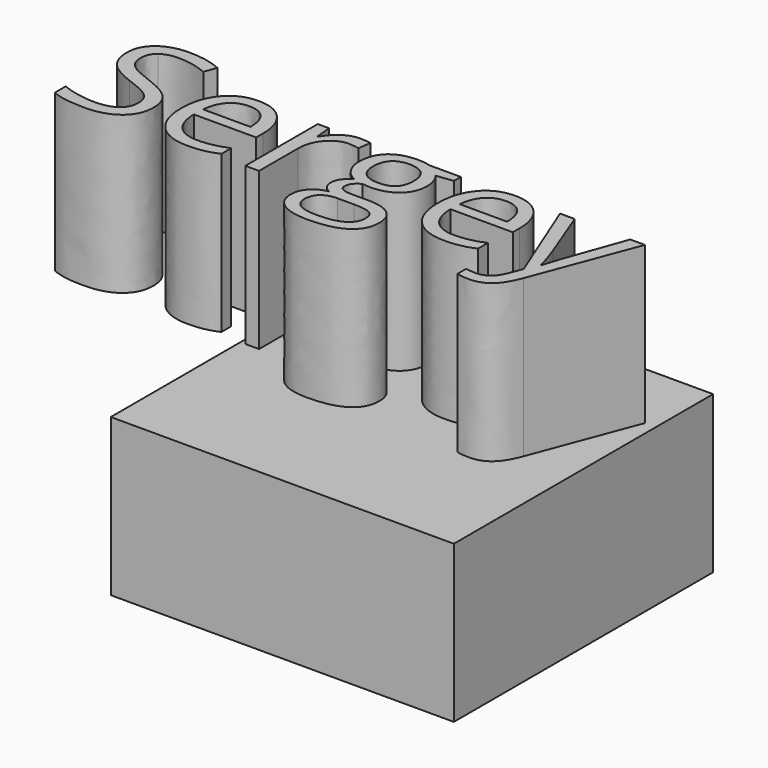
from build123d import *

# Parameters (mm, degrees)
F0_W         = 55.5511265993
F0_H         = 52.472114563
F1_DEPTH     = 25.4
F2_TEXT_SIZE = 27.3882670121
F4_DEPTH     = 25.4
F6_DEPTH     = 25.4


# Not quite as in the source:
# - Text() gives the source's letters only with a copy of the font that has no kerning and outlines rounded to 1/6400 em; it was checked with that copy


with BuildPart() as f1:
    # F0 (on Top) → F1 (new body)
    with BuildSketch(Plane.XY):
        with Locations((3.0288919806, -4.1702836752)):
            Rectangle(F0_W, F0_H)
    extrude(amount=F1_DEPTH)

    # F2 (on face) → F4 (join)
    with BuildSketch(Plane.XY.offset(25.4)):
        with Locations((-56.7010578234, -4.1702836752)):
            Text('Sergey', F2_TEXT_SIZE, font='Open Sans', text_align=(TextAlign.LEFT, TextAlign.BOTTOM))
    extrude(amount=F4_DEPTH)

    # F3 (on face) → F6 (join)
    with BuildSketch(Plane.XY.offset(25.4)):
        with BuildLine():
            add(Edge.make_bspline(
                [(-42.981247817, 1.0334870571), (-42.981247817, -1.5470012254), (-44.8534926323, -2.993444077)],
                knots=[0, 0, 0, 1, 1, 1], degree=2))
            add(Edge.make_bspline(
                [(-44.1366903316, 4.2944025982), (-42.981247817, 3.0362540824), (-42.981247817, 1.0334870571)],
                knots=[0, 0, 0, 1, 1, 1], degree=2))
            add(Edge.make_bspline(
                [(-48.3690334683, 6.6480817946), (-45.2921328461, 5.5525511141), (-44.1366903316, 4.2944025982)],
                knots=[0, 0, 0, 1, 1, 1], degree=2))
            add(Edge.make_bspline(
                [(-51.0907425026, 7.844178768), (-50.2006238247, 7.3028325528), (-48.3690334683, 6.6480817946)],
                knots=[0, 0, 0, 1, 1, 1], degree=2))
            add(Edge.make_bspline(
                [(-52.3553101436, 9.0359963247), (-51.9808611805, 8.3855249832), (-51.0907425026, 7.844178768)],
                knots=[0, 0, 0, 1, 1, 1], degree=2))
            add(Edge.make_bspline(
                [(-52.7297591066, 10.700689429), (-52.7297591066, 9.6864676662), (-52.3553101436, 9.0359963247)],
                knots=[0, 0, 0, 1, 1, 1], degree=2))
            add(Edge.make_bspline(
                [(-51.7133976355, 12.8532360395), (-52.7297591066, 12.0786616131), (-52.7297591066, 10.700689429)],
                knots=[0, 0, 0, 1, 1, 1], degree=2))
            add(Edge.make_bspline(
                [(-48.8911223082, 13.627810466), (-50.6970361643, 13.627810466), (-51.7133976355, 12.8532360395)],
                knots=[0, 0, 0, 1, 1, 1], degree=2))
            add(Edge.make_bspline(
                [(-44.1837639155, 12.6135887032), (-46.6059137794, 13.627810466), (-48.8911223082, 13.627810466)],
                knots=[0, 0, 0, 1, 1, 1], degree=2))
            Line((-44.1837639155, 12.6135887032), (-43.4733807399, 14.5906792281))
            add(Edge.make_bspline(
                [(-48.8354898908, 15.6605334083), (-45.9212071041, 15.6605334083), (-43.4733807399, 14.5906792281)],
                knots=[0, 0, 0, 1, 1, 1], degree=2))
            add(Edge.make_bspline(
                [(-53.3310171559, 14.3232156831), (-51.6342284261, 15.6605334083), (-48.8354898908, 15.6605334083)],
                knots=[0, 0, 0, 1, 1, 1], degree=2))
            add(Edge.make_bspline(
                [(-55.0278058856, 10.7263659294), (-55.0278058856, 12.9858979579), (-53.3310171559, 14.3232156831)],
                knots=[0, 0, 0, 1, 1, 1], degree=2))
            add(Edge.make_bspline(
                [(-53.8573854125, 7.2365015937), (-55.0278058856, 8.5738193189), (-55.0278058856, 10.7263659294)],
                knots=[0, 0, 0, 1, 1, 1], degree=2))
            add(Edge.make_bspline(
                [(-49.9609764884, 4.9234768562), (-52.6869649394, 5.8991838685), (-53.8573854125, 7.2365015937)],
                knots=[0, 0, 0, 1, 1, 1], degree=2))
            add(Edge.make_bspline(
                [(-47.0531128267, 3.6803062988), (-48.0095624638, 4.2302113474), (-49.9609764884, 4.9234768562)],
                knots=[0, 0, 0, 1, 1, 1], degree=2))
            add(Edge.make_bspline(
                [(-45.6879788928, 2.482069617), (-46.0966631896, 3.1304012502), (-47.0531128267, 3.6803062988)],
                knots=[0, 0, 0, 1, 1, 1], degree=2))
            add(Edge.make_bspline(
                [(-45.279294596, 0.8195162211), (-45.279294596, 1.8337379839), (-45.6879788928, 2.482069617)],
                knots=[0, 0, 0, 1, 1, 1], degree=2))
            add(Edge.make_bspline(
                [(-46.4304576938, -1.5833762676), (-45.279294596, -0.7210737984), (-45.279294596, 0.8195162211)],
                knots=[0, 0, 0, 1, 1, 1], degree=2))
            add(Edge.make_bspline(
                [(-49.8539910703, -2.4456787368), (-47.5816207917, -2.4456787368), (-46.4304576938, -1.5833762676)],
                knots=[0, 0, 0, 1, 1, 1], degree=2))
            add(Edge.make_bspline(
                [(-52.6612884391, -2.1503989831), (-51.2448015046, -2.4456787368), (-49.8539910703, -2.4456787368)],
                knots=[0, 0, 0, 1, 1, 1], degree=2))
            add(Edge.make_bspline(
                [(-55.2845708888, -1.3501480563), (-54.0777753736, -1.8551192293), (-52.6612884391, -2.1503989831)],
                knots=[0, 0, 0, 1, 1, 1], degree=2))
            Line((-55.2845708888, -1.3501480563), (-55.2845708888, -3.5412094173))
            add(Edge.make_bspline(
                [(-49.935299988, -4.4398869286), (-53.4101863652, -4.4398869286), (-55.2845708888, -3.5412094173)],
                knots=[0, 0, 0, 1, 1, 1], degree=2))
            add(Edge.make_bspline(
                [(-44.8534926323, -2.993444077), (-46.7257374476, -4.4398869286), (-49.935299988, -4.4398869286)],
                knots=[0, 0, 0, 1, 1, 1], degree=2))
        make_face()
    extrude(amount=F6_DEPTH)


solid = f1.part
